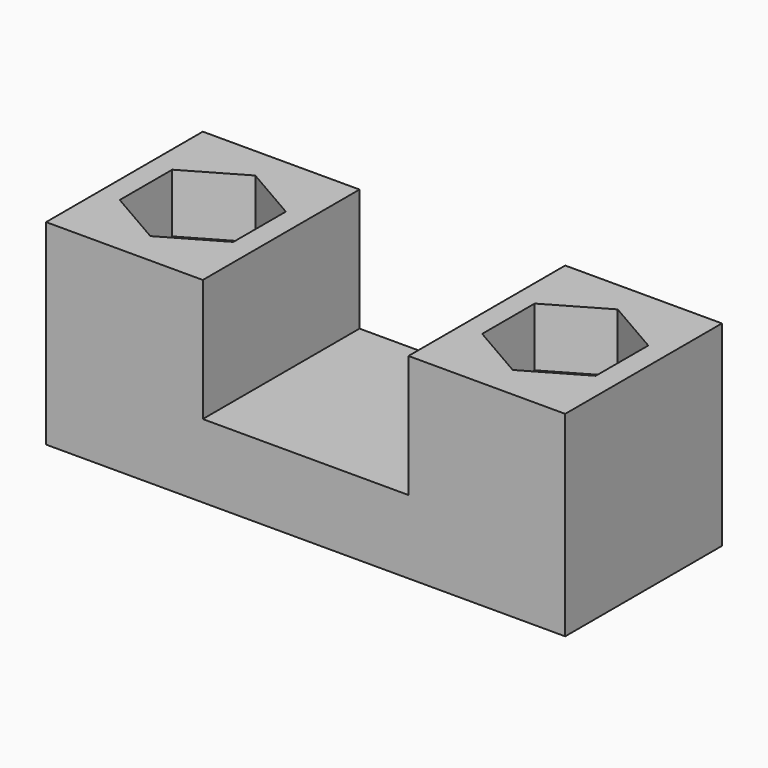
from build123d import *

# Parameters (mm, degrees)
F1_DEPTH = 10
F3_DEPTH = 10.001
F4_DEPTH = 3


# Not quite as in the source:
# - a pattern or mirror of a feature is missing from the dataset's text; its kind, count and spacing are read off the source's solid


with BuildPart() as f1:
    # F0 (on Front) → F1 (new body)
    with BuildSketch(Plane.XZ):
        Polygon((0, -10), (0, -6.25), (-5.25, -6.25), (-5.25, 0), (-13.25, 0), (-13.25, -10), align=None)
        Polygon((5.25, -6.25), (0, -6.25), (0, -10), (13.25, -10), (13.25, 0), (5.25, 0), align=None)
    extrude(amount=F1_DEPTH)

    # F2 (on face) → F3 (cut, through all)
    with BuildSketch(Plane.XY):
        with BuildLine():
            ThreePointArc((-9.25, -3.3), (-10.452081528, -3.797918472), (-10.95, -5))
            Line((-10.95, -5), (-9.25, -5))
            Line((-9.25, -5), (-9.25, -3.3))
        make_face()
        with BuildLine():
            Line((-9.25, -3.3), (-9.25, -5))
            Line((-9.25, -5), (-7.55, -5))
            ThreePointArc((-7.55, -5), (-8.047918472, -3.797918472), (-9.25, -3.3))
        make_face()
        with BuildLine():
            Line((-7.55, -5), (-9.25, -5))
            Line((-9.25, -5), (-9.25, -6.7))
            ThreePointArc((-9.25, -6.7), (-8.047918472, -6.202081528), (-7.55, -5))
        make_face()
        with BuildLine():
            Line((-9.25, -5), (-10.95, -5))
            ThreePointArc((-10.95, -5), (-10.452081528, -6.202081528), (-9.25, -6.7))
            Line((-9.25, -6.7), (-9.25, -5))
        make_face()
    f3 = extrude(amount=-F3_DEPTH, mode=Mode.SUBTRACT)

    # F3_copies: F3 across plane
    add(f3.mirror(Plane(origin=(0, 0, 0), x_dir=(0, 0, 1), z_dir=(1, 0, 0))), mode=Mode.SUBTRACT)

    # F2 (on face) → F4 (cut)
    with BuildSketch(Plane.XY):
        with BuildLine():
            Line((-12.15, -3.3256842194), (-12.15, -5))
            Line((-12.15, -5), (-10.95, -5))
            ThreePointArc((-10.95, -5), (-10.452081528, -3.797918472), (-9.25, -3.3))
            Line((-9.25, -3.3), (-9.25, -1.6513684387))
            Line((-9.25, -1.6513684387), (-12.15, -3.3256842194))
        make_face()
        with BuildLine():
            Line((-10.95, -5), (-12.15, -5))
            Line((-12.15, -5), (-12.15, -6.6743157806))
            Line((-12.15, -6.6743157806), (-9.25, -8.3486315613))
            Line((-9.25, -8.3486315613), (-9.25, -6.7))
            ThreePointArc((-9.25, -6.7), (-10.452081528, -6.202081528), (-10.95, -5))
        make_face()
        with BuildLine():
            Line((-9.25, -1.6513684387), (-9.25, -3.3))
            ThreePointArc((-9.25, -3.3), (-8.047918472, -3.797918472), (-7.55, -5))
            Line((-7.55, -5), (-6.35, -5))
            Line((-6.35, -5), (-6.35, -3.3256842194))
            Line((-6.35, -3.3256842194), (-9.25, -1.6513684387))
        make_face()
        with BuildLine():
            ThreePointArc((-7.55, -5), (-8.047918472, -6.202081528), (-9.25, -6.7))
            Line((-9.25, -6.7), (-9.25, -8.3486315613))
            Line((-9.25, -8.3486315613), (-6.35, -6.6743157806))
            Line((-6.35, -6.6743157806), (-6.35, -5))
            Line((-6.35, -5), (-7.55, -5))
        make_face()
    f4 = extrude(amount=-F4_DEPTH, mode=Mode.SUBTRACT)

    # F4_copies: F4 across plane
    add(f4.mirror(Plane(origin=(0, 0, 0), x_dir=(0, 0, 1), z_dir=(1, 0, 0))), mode=Mode.SUBTRACT)


solid = f1.part
